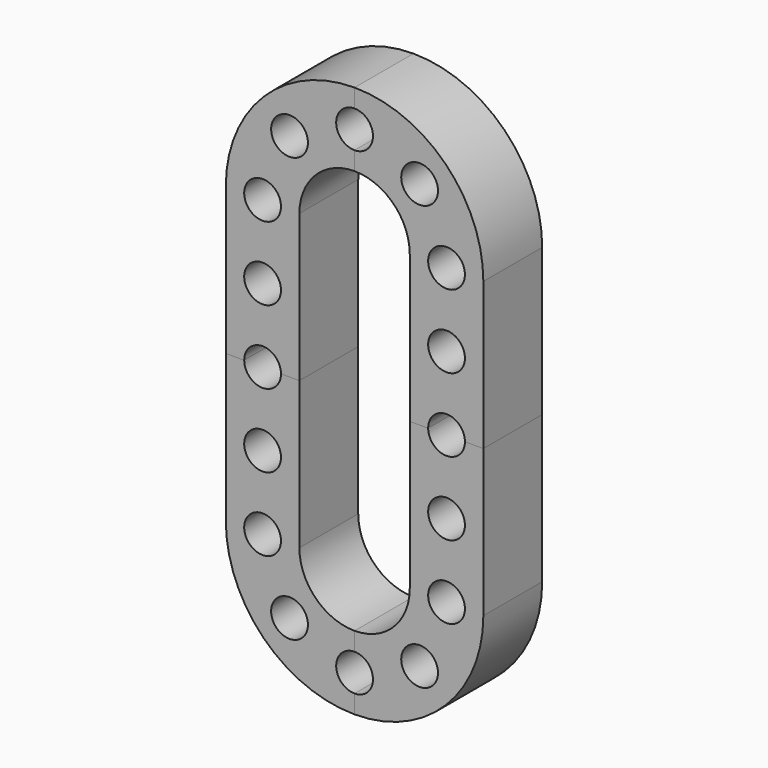
from build123d import *
from build123d import SkipClean  # not in build123d's __all__

# Parameters (mm, degrees)
F0_R     = 5
F1_DEPTH = 20


with BuildPart() as f1:
    # F0 (on Front) → F1 (new body)
    with BuildSketch(Plane.XZ):
        with BuildLine():
            Line((-15, 0), (-15, 40))
            ThreePointArc((-15, 40), (-10.6066017178, 50.6066017178), (0, 55))
            Line((0, 55), (0, 60))
            ThreePointArc((0, 60), (-5, 65), (0, 70))
            Line((0, 70), (0, 75))
            ThreePointArc((0, 75), (-24.7487373415, 64.7487373415), (-35, 40))
            Line((-35, 40), (-35, 0))
            Line((-35, 0), (-30, 0))
            ThreePointArc((-30, 0), (-25, 5), (-20, 0))
            Line((-20, 0), (-15, 0))
        make_face()
        with Locations((-25, 20)):
            Circle(F0_R, mode=Mode.SUBTRACT)
        with Locations((-25, 40)):
            Circle(F0_R, mode=Mode.SUBTRACT)
        with Locations((-17.6776695297, 57.6776695297)):
            Circle(F0_R, mode=Mode.SUBTRACT)
    extrude(amount=F1_DEPTH)

    # F2: F1 across plane


with BuildPart() as f1_1:
    add(f1.part, clean=False)
    with SkipClean():  # cleaning this boolean's faces spoils the solid; the shape is the same uncleaned
        add(f1.part.mirror(Plane.YZ), clean=False)

    # F3: F1 across plane


with BuildPart() as f1_2:
    add(f1_1.part, clean=False)
    with SkipClean():  # cleaning this boolean's faces spoils the solid; the shape is the same uncleaned
        add(f1_1.part.mirror(Plane.XY), clean=False)


solid = f1_2.part
